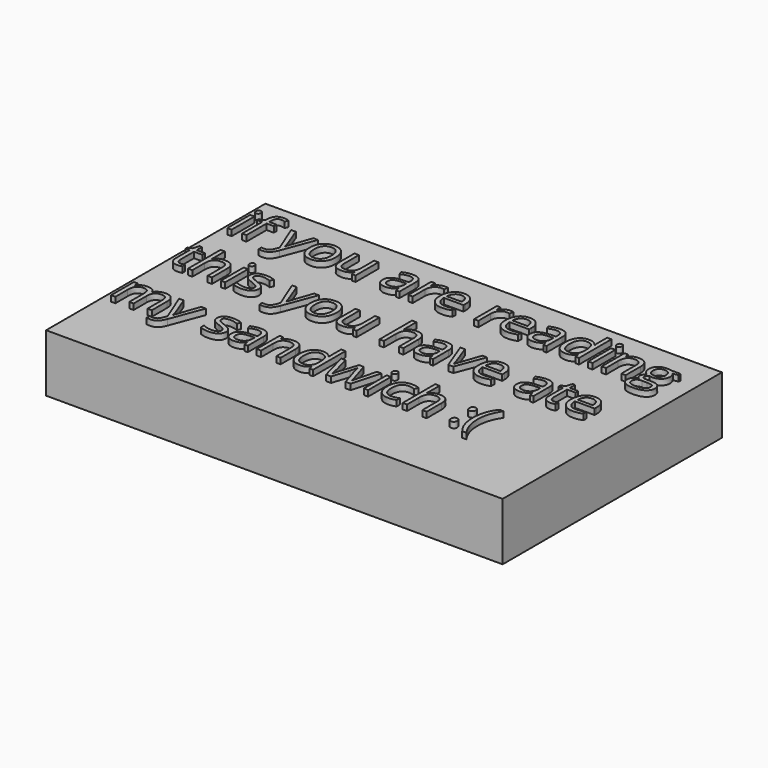
from build123d import *

# Parameters (mm, degrees)
F0_W         = 201.20742172
F0_H         = 120.803270489
F1_DEPTH     = 25.4
F2_TEXT_SIZE = 23.5387874353
F3_DEPTH     = 2.54
F5_DEPTH     = 15.24


# Not quite as in the source:
# - Text() gives the source's letters only with a copy of the font that has no kerning and outlines rounded to 1/6400 em; it was checked with that copy


with BuildPart() as f1:
    # F0 (on Top) → F1 (new body)
    with BuildSketch(Plane.XY):
        with Locations((5.7150013745, -10.247586295)):
            Rectangle(F0_W, F0_H)
    extrude(amount=F1_DEPTH)

    # F2 (on face) → F3 (join)
    with BuildSketch(Plane.XY.offset(25.4)):
        with Locations((-92.7209481597, 23.9438805729)):
            Text('if you are reading', F2_TEXT_SIZE, font='Open Sans', text_align=(TextAlign.LEFT, TextAlign.BOTTOM))
        with Locations((-92.7209481597, -8.0688703391)):
            Text('this you have ate', F2_TEXT_SIZE, font='Open Sans', text_align=(TextAlign.LEFT, TextAlign.BOTTOM))
        with Locations((-92.7209481597, -40.0816212512)):
            Text('my sandwich :(', F2_TEXT_SIZE, font='Open Sans', text_align=(TextAlign.LEFT, TextAlign.BOTTOM))
    extrude(amount=F3_DEPTH)

    # F4 (on face) → F5 (join)
    with BuildSketch(Plane(origin=(0, 0, 0), x_dir=(1, 0, 0), z_dir=(0, 0, -1))):
        Polygon((-9.7573117879, 30.3522876159), (-15.127589931, 12.2723482119), (0.4079470427, 1.5779016565), (15.379715069, 13.0483095985), (9.0972396072, 30.8318581268), align=None)
    extrude(amount=F5_DEPTH)


solid = f1.part
